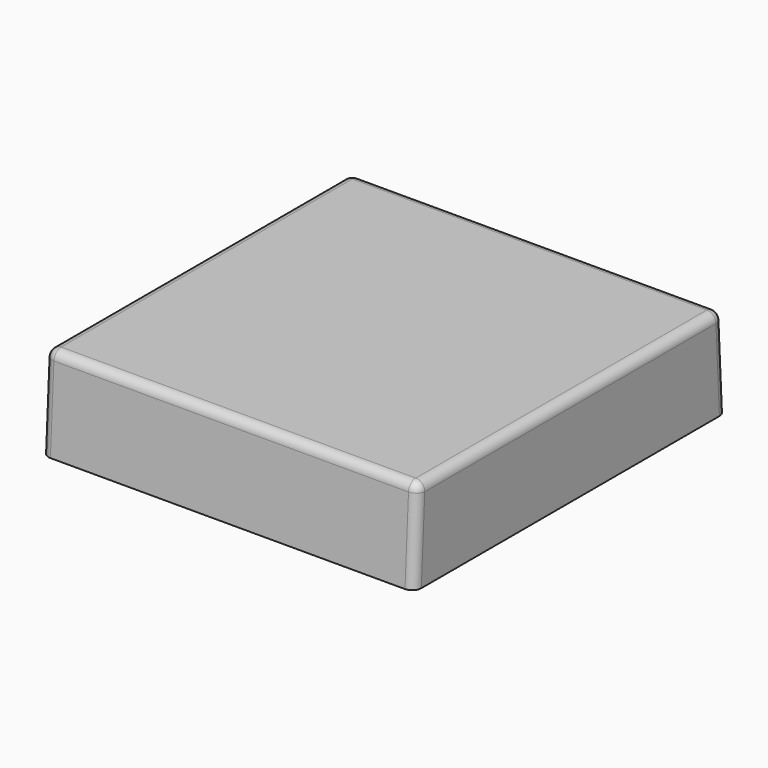
from build123d import *

# Parameters (mm, degrees)
F3_DEPTH      = 51.5
F3_DEPTH_BACK = 51.5
F4_R          = 2.5
F5_T          = -2


with BuildPart() as f3:
    # F2 (on Right) → F3 (new body, two sides)
    with BuildSketch(Plane.YZ) as f3_sk:
        Polygon((-54, 0), (54, 0), (52.6636016283, 25.5), (-52.6636016283, 25.5), align=None)
    extrude(amount=F3_DEPTH)
    extrude(f3_sk.sketch, amount=-F3_DEPTH_BACK)

    # F4
    f4_edges = [f3.edges().sort_by_distance(p)[0] for p in [
        (0, -52.663602, 25.5),
        (-51.5, -53.331801, 12.75),
        (-51.5, 0, 25.5),
        (51.5, 0, 25.5),
        (51.5, -53.331801, 12.75),
        (51.5, 53.331801, 12.75),
        (0, 52.663602, 25.5),
        (-51.5, 53.331801, 12.75),
    ]]
    fillet(f4_edges, radius=F4_R)

    # F5
    f5_openings = [f3.faces().sort_by_distance(p)[0] for p in [
        (0, 0, 0),
    ]]
    offset(amount=F5_T, openings=f5_openings, kind=Kind.INTERSECTION)


solid = f3.part
